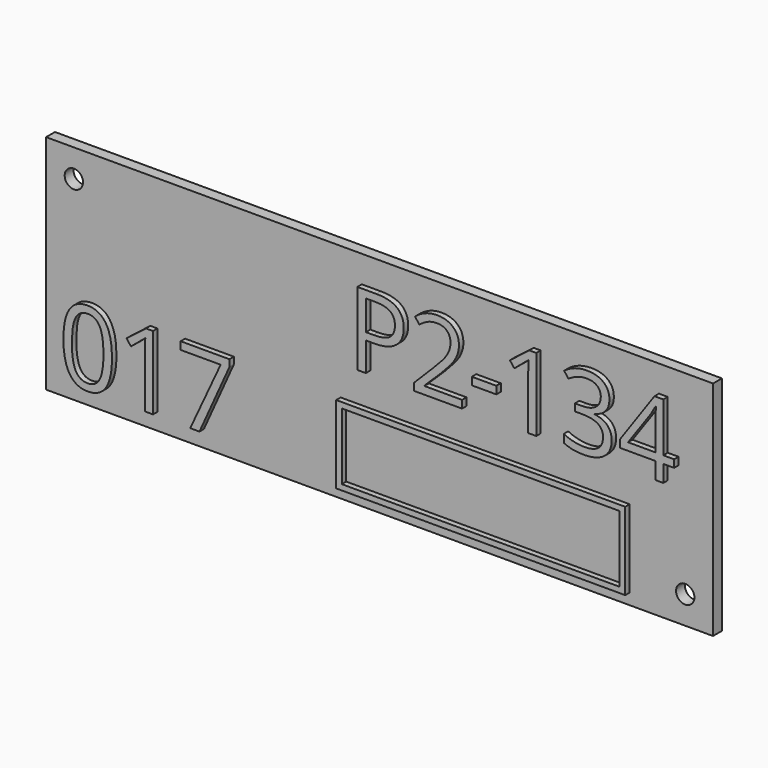
from build123d import *

# Parameters (mm, degrees)
F0_W         = 120
F0_H         = 40
F1_DEPTH     = 2
F3_D         = 3.3
F4_TEXT_SIZE = 18.430525558
F5_DEPTH     = 1
F6_TEXT_SIZE = 18.5054667028
F7_DEPTH     = 1
F8_W         = 52
F8_H         = 14
F8_W_2       = 49.99999962
F8_H_2       = 11.99999962
F9_DEPTH     = 1


# Not quite as in the source:
# - Text() gives the source's letters only with a copy of the font that has no kerning and outlines rounded to 1/6400 em; it was checked with that copy


with BuildPart() as f1:
    # F0 (on Front) → F1 (new body)
    with BuildSketch(Plane.XZ):
        Rectangle(F0_W, F0_H)
    extrude(amount=F1_DEPTH)

    # F3 (through all)
    with Locations(Plane.XZ.offset(2)):
        with Locations((-55, 15), (55, -15)):
            Hole(F3_D / 2)

    # F4 (on face) → F5 (join)
    with BuildSketch(Plane.XZ.offset(2)):
        with Locations((-5, 2)):
            Text('P2-134', F4_TEXT_SIZE, font='Open Sans', text_align=(TextAlign.LEFT, TextAlign.BOTTOM))
    extrude(amount=F5_DEPTH)

    # F6 (on face) → F7 (join)
    with BuildSketch(Plane.XZ.offset(2)):
        with Locations((-57, -17)):
            Text('017', F6_TEXT_SIZE, font='Open Sans', text_align=(TextAlign.LEFT, TextAlign.BOTTOM))
    extrude(amount=F7_DEPTH)

    # F8 (on face) → F9 (join)
    with BuildSketch(Plane.XZ.offset(2)):
        with Locations((19, -11)):
            Rectangle(F8_W, F8_H)
        with Locations((19, -11)):
            Rectangle(F8_W_2, F8_H_2, mode=Mode.SUBTRACT)
    extrude(amount=F9_DEPTH)


solid = f1.part
